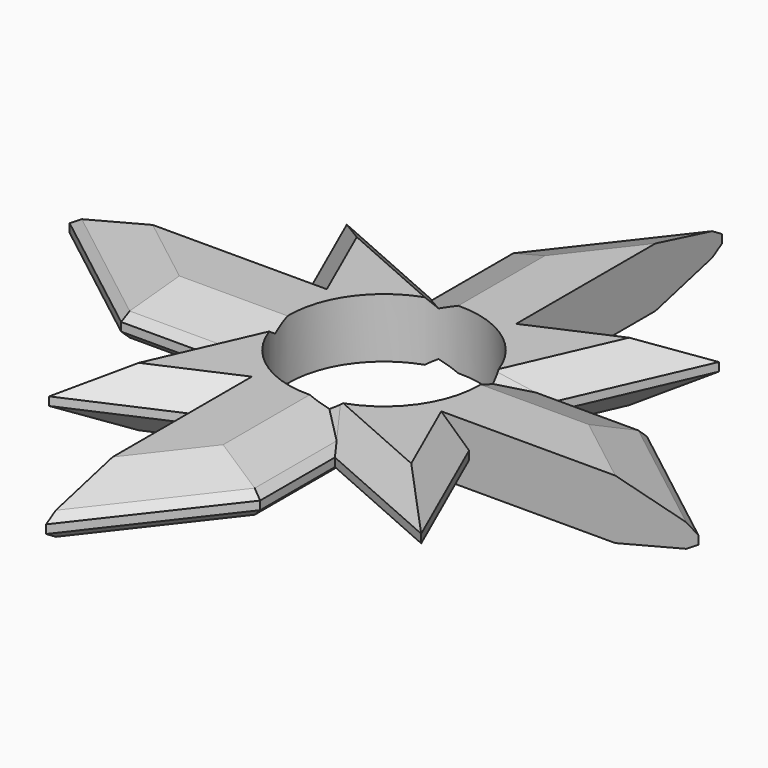
from build123d import *

# Parameters (mm, degrees)
F1_DEPTH      = 7
F2_T1_DEPTH   = 35.6796346597
F2_T3_DEPTH   = 35.6796346597
F2_T5_DEPTH   = 35.6796346597
F2_T7_DEPTH   = 35.6796346597
F2_T12_DEPTH  = 26.4420979278
F2_T17_DEPTH  = 26.4420979278
F2_T22_DEPTH  = 26.4420979278
F2_T27_DEPTH  = 26.4420979278
F2_T32_DEPTH  = 32.5914188112
F2_T37_DEPTH  = 32.5914188112
F2_T42_DEPTH  = 32.5914188112
F2_T47_DEPTH  = 32.5914188112
F2_T52_DEPTH  = 32.5914188112
F2_T57_DEPTH  = 32.5914188112
F2_T62_DEPTH  = 32.5914188112
F2_T67_DEPTH  = 32.5914188112
F2_T72_DEPTH  = 26.4420979278
F2_T77_DEPTH  = 32.5914188112
F2_T82_DEPTH  = 32.5914188112
F2_T87_DEPTH  = 26.4420979278
F2_T92_DEPTH  = 32.5914188112
F2_T97_DEPTH  = 32.5914188112
F2_T102_DEPTH = 26.4420979278
F2_T107_DEPTH = 32.5914188112
F2_T112_DEPTH = 32.5914188112
F2_T117_DEPTH = 26.4420979278
F2_T122_DEPTH = 32.5914188112
F2_T127_DEPTH = 32.5914188112
F2_T133_DEPTH = 26.4420979278
F2_T137_DEPTH = 32.5914188112
F2_T144_DEPTH = 26.4420979278
F2_T148_DEPTH = 32.5914188112
F2_T155_DEPTH = 26.4420979278
F2_T159_DEPTH = 32.5914188112
F2_T166_DEPTH = 26.4420979278
F2_T170_DEPTH = 32.5914188112
F2_T177_DEPTH = 26.4420979278
F2_T181_DEPTH = 32.5914188112
F2_T188_DEPTH = 26.4420979278
F2_T192_DEPTH = 32.5914188112
F2_T199_DEPTH = 26.4420979278
F2_T203_DEPTH = 32.5914188112
F2_T210_DEPTH = 26.4420979278
F2_T214_DEPTH = 32.5914188112
F3_T1_DEPTH   = 30.9109915853
F3_T3_DEPTH   = 30.9109915853
F3_T5_DEPTH   = 30.9109915853
F3_T7_DEPTH   = 30.9109915853
F3_T12_DEPTH  = 29.7913643174
F3_T17_DEPTH  = 29.7913643174
F3_T22_DEPTH  = 29.7913643174
F3_T27_DEPTH  = 29.7913643174
F3_T32_DEPTH  = 29.7913643174
F3_T37_DEPTH  = 29.7913643174
F3_T42_DEPTH  = 29.7913643174
F3_T47_DEPTH  = 29.7913643174


# Not quite as in the source:
# - a fillet or chamfer that OpenCascade refuses, or shapes differently, is made with other operations: its cross-section is extruded or revolved along the edge and cut away or added


with BuildPart() as f1:
    # F0 (on Top) → F1 (new body)
    with BuildSketch(Plane.XY):
        Polygon((-6.2057178847, 25.9939282815), (6.2057178847, 25.9939282815), (6.2057178847, 41.9939282815), align=None)
        Polygon((-6.2057178847, 25.9939282815), (-6.2057178847, 14.9819282815), (6.2057178847, 25.9939282815), align=None)
        Polygon((6.2057178847, 25.9939282815), (-6.2057178847, 14.9819282815), (6.2057178847, 14.9819282815), align=None)
        Polygon((21.9075315821, 21.9075315821), (6.2057178847, 14.9819282815), (10.5938230831, 10.5938230831), align=None)
        Polygon((21.9075315821, 21.9075315821), (10.5938230831, 10.5938230831), (14.9819282815, 6.2057178847), align=None)
        Polygon((25.9939282815, 6.2057178847), (14.9819282815, 6.2057178847), (25.9939282815, -6.2057178847), align=None)
        Polygon((14.9819282815, 6.2057178847), (14.9819282815, -6.2057178847), (25.9939282815, -6.2057178847), align=None)
        Polygon((25.9939282815, 6.2057178847), (25.9939282815, -6.2057178847), (41.9939282815, -6.2057178847), align=None)
        Polygon((10.5938230831, -10.5938230831), (6.2057178847, -14.9819282815), (21.9075315821, -21.9075315821), align=None)
        Polygon((-14.9819282815, 6.2057178847), (-14.9819282815, 0), (-14.9819282815, -6.2057178847), (-10.5938230831, -10.5938230831), (-6.2057178847, -14.9819282815), (6.2057178847, -14.9819282815), (10.5938230831, -10.5938230831), (14.9819282815, -6.2057178847), (14.9819282815, 6.2057178847), (10.5938230831, 10.5938230831), (6.2057178847, 14.9819282815), (-6.2057178847, 14.9819282815), (-10.5938230831, 10.5938230831), align=None)
        with BuildLine():
            ThreePointArc((-11.2, 0), (0, 11.2), (11.2, 0))
            ThreePointArc((11.2, 0), (0, -11.2), (-11.2, 0))
        make_face(mode=Mode.SUBTRACT)
        Polygon((-25.9939282815, -6.2057178847), (-25.9939282815, 6.2057178847), (-41.9939282815, 6.2057178847), align=None)
        Polygon((-25.9939282815, -6.2057178847), (-14.9819282815, -6.2057178847), (-25.9939282815, 6.2057178847), align=None)
        Polygon((-14.9819282815, -6.2057178847), (-14.9819282815, 0), (-14.9819282815, 6.2057178847), (-25.9939282815, 6.2057178847), align=None)
        Polygon((-21.9075315821, 21.9075315821), (-14.9819282815, 6.2057178847), (-10.5938230831, 10.5938230831), align=None)
        Polygon((-21.9075315821, 21.9075315821), (-10.5938230831, 10.5938230831), (-6.2057178847, 14.9819282815), align=None)
        Polygon((6.2057178847, -25.9939282815), (6.2057178847, -14.9819282815), (-6.2057178847, -25.9939282815), align=None)
        Polygon((6.2057178847, -25.9939282815), (-6.2057178847, -25.9939282815), (-6.2057178847, -41.9939282815), align=None)
        Polygon((6.2057178847, -14.9819282815), (-6.2057178847, -14.9819282815), (-6.2057178847, -25.9939282815), align=None)
        Polygon((-6.2057178847, -14.9819282815), (-10.5938230831, -10.5938230831), (-21.9075315821, -21.9075315821), align=None)
        Polygon((-10.5938230831, -10.5938230831), (-14.9819282815, -6.2057178847), (-21.9075315821, -21.9075315821), align=None)
        Polygon((14.9819282815, -6.2057178847), (10.5938230831, -10.5938230831), (21.9075315821, -21.9075315821), align=None)
    extrude(amount=F1_DEPTH)

    # F2: chamfer of 3 on 32 edges, made by hand

    # F2_s2 → F2_t1 (cut)
    with BuildSketch(Plane(origin=(27.3976190365, 35.3191937444, 0), x_dir=(0, 0, 1), z_dir=(-0.6129244305, -0.7901415332, 0))):
        Polygon((4, 20.8357091325), (7, 17.8357091325), (7, 20.8357091325), align=None)
        Polygon((3, 20.8357091325), (0, 17.8357091325), (0, 20.8357091325), align=None)
    extrude(amount=F2_T1_DEPTH, mode=Mode.SUBTRACT)

    # F2_s4 → F2_t3 (cut)
    with BuildSketch(Plane(origin=(-35.3191937444, 27.3976190365, 0), x_dir=(0, 0, 1), z_dir=(0.7901415332, -0.6129244305, 0))):
        Polygon((4, 20.8357091325), (7, 17.8357091325), (7, 20.8357091325), align=None)
        Polygon((3, 20.8357091325), (0, 17.8357091325), (0, 20.8357091325), align=None)
    extrude(amount=F2_T3_DEPTH, mode=Mode.SUBTRACT)

    # F2_s6 → F2_t5 (cut)
    with BuildSketch(Plane(origin=(-27.3976190365, -35.3191937444, 0), x_dir=(0, 0, 1), z_dir=(0.6129244305, 0.7901415332, 0))):
        Polygon((4, 20.8357091325), (7, 17.8357091325), (7, 20.8357091325), align=None)
        Polygon((3, 20.8357091325), (0, 17.8357091325), (0, 20.8357091325), align=None)
    extrude(amount=F2_T5_DEPTH, mode=Mode.SUBTRACT)

    # F2_s8 → F2_t7 (cut)
    with BuildSketch(Plane(origin=(35.3191937444, -27.3976190365, 0), x_dir=(0, 0, 1), z_dir=(-0.7901415332, 0.6129244305, 0))):
        Polygon((4, 20.8357091325), (7, 17.8357091325), (7, 20.8357091325), align=None)
        Polygon((3, 20.8357091325), (0, 17.8357091325), (0, 20.8357091325), align=None)
    extrude(amount=F2_T7_DEPTH, mode=Mode.SUBTRACT)


with BuildPart() as f2_tool10:
    # F2_s11 → F2_t12 (new body)
    with BuildSketch(Plane.YZ.offset(33.7089772454)):
        Polygon((6.2057178847, 4), (3.2057178847, 7), (6.2057178847, 7), align=None)
    extrude(amount=-F2_T12_DEPTH)

    split(bisect_by=Plane(origin=(10.2505901429, -4.5212306231, 0), x_dir=(0, 0, 1), z_dir=(0.9149536801, -0.4035588722, 0)), keep=Keep.TOP)


with BuildPart() as f1_1:
    add(f1.part)

    # F2_t9: cut F2_tool10
    add(f2_tool10.part, mode=Mode.SUBTRACT)


with BuildPart() as f2_tool15:
    # F2_s16 → F2_t17 (new body)
    with BuildSketch(Plane.XZ.offset(33.7089772454)):
        Polygon((6.2057178847, 4), (3.2057178847, 7), (6.2057178847, 7), align=None)
    extrude(amount=-F2_T17_DEPTH)

    split(bisect_by=Plane(origin=(-4.5212306231, -10.2505901429, 0), x_dir=(0, 0, 1), z_dir=(-0.4035588722, -0.9149536801, 0)), keep=Keep.TOP)


with BuildPart() as f1_2:
    add(f1_1.part)

    # F2_t14: cut F2_tool15
    add(f2_tool15.part, mode=Mode.SUBTRACT)


with BuildPart() as f2_tool20:
    # F2_s21 → F2_t22 (new body)
    with BuildSketch(Plane.YZ.offset(-33.7089772454)):
        Polygon((-6.2057178847, 4), (-3.2057178847, 7), (-6.2057178847, 7), align=None)
    extrude(amount=F2_T22_DEPTH)

    split(bisect_by=Plane(origin=(-10.2505901429, 4.5212306231, 0), x_dir=(0, 0, 1), z_dir=(-0.9149536801, 0.4035588722, 0)), keep=Keep.TOP)


with BuildPart() as f1_3:
    add(f1_2.part)

    # F2_t19: cut F2_tool20
    add(f2_tool20.part, mode=Mode.SUBTRACT)


with BuildPart() as f2_tool25:
    # F2_s26 → F2_t27 (new body)
    with BuildSketch(Plane.XZ.offset(-33.7089772454)):
        Polygon((-6.2057178847, 4), (-3.2057178847, 7), (-6.2057178847, 7), align=None)
    extrude(amount=F2_T27_DEPTH)

    split(bisect_by=Plane(origin=(4.5212306231, 10.2505901429, 0), x_dir=(0, 0, 1), z_dir=(0.4035588722, 0.9149536801, 0)), keep=Keep.TOP)


with BuildPart() as f1_4:
    add(f1_3.part)

    # F2_t24: cut F2_tool25
    add(f2_tool25.part, mode=Mode.SUBTRACT)


with BuildPart() as f2_tool30:
    # F2_s31 → F2_t32 (new body)
    with BuildSketch(Plane(origin=(-3.6680360663, 1.61786168, 0), x_dir=(0, 0, 1), z_dir=(-0.9149536801, 0.4035588722, 0))):
        Polygon((4, 11.2033979054), (7, 8.2033979054), (7, 11.2033979054), align=None)
    extrude(amount=F2_T32_DEPTH)

    split(bisect_by=Plane.YZ.offset(-6.2057178847), keep=Keep.BOTTOM)


with BuildPart() as f1_5:
    add(f1_4.part)

    # F2_t29: cut F2_tool30
    add(f2_tool30.part, mode=Mode.SUBTRACT)


with BuildPart() as f2_tool35:
    # F2_s36 → F2_t37 (new body)
    with BuildSketch(Plane(origin=(-14.7704178977, 33.4876746467, 0), x_dir=(0, 0, 1), z_dir=(0.4035588722, -0.9149536801, 0))):
        Polygon((4, 11.2033979054), (7, 8.2033979054), (7, 11.2033979054), align=None)
    extrude(amount=F2_T37_DEPTH)

    split(bisect_by=Plane.XZ.offset(-6.2057178847), keep=Keep.BOTTOM)


with BuildPart() as f1_6:
    add(f1_5.part)

    # F2_t34: cut F2_tool35
    add(f2_tool35.part, mode=Mode.SUBTRACT)


with BuildPart() as f2_tool40:
    # F2_s41 → F2_t42 (new body)
    with BuildSketch(Plane(origin=(33.4876746467, 14.7704178977, 0), x_dir=(0, 0, 1), z_dir=(-0.9149536801, -0.4035588722, 0))):
        Polygon((4, 11.2033979054), (7, 8.2033979054), (7, 11.2033979054), align=None)
    extrude(amount=F2_T42_DEPTH)

    split(bisect_by=Plane.YZ.offset(6.2057178847), keep=Keep.TOP)


with BuildPart() as f1_7:
    add(f1_6.part)

    # F2_t39: cut F2_tool40
    add(f2_tool40.part, mode=Mode.SUBTRACT)


with BuildPart() as f2_tool45:
    # F2_s46 → F2_t47 (new body)
    with BuildSketch(Plane(origin=(1.61786168, 3.6680360663, 0), x_dir=(0, 0, 1), z_dir=(0.4035588722, 0.9149536801, 0))):
        Polygon((4, 11.2033979054), (7, 8.2033979054), (7, 11.2033979054), align=None)
    extrude(amount=F2_T47_DEPTH)

    split(bisect_by=Plane.XZ.offset(-6.2057178847), keep=Keep.BOTTOM)


with BuildPart() as f1_8:
    add(f1_7.part)

    # F2_t44: cut F2_tool45
    add(f2_tool45.part, mode=Mode.SUBTRACT)


with BuildPart() as f2_tool50:
    # F2_s51 → F2_t52 (new body)
    with BuildSketch(Plane(origin=(-1.61786168, -3.6680360663, 0), x_dir=(0, 0, 1), z_dir=(-0.4035588722, -0.9149536801, 0))):
        Polygon((4, 11.2033979054), (7, 8.2033979054), (7, 11.2033979054), align=None)
    extrude(amount=F2_T52_DEPTH)

    split(bisect_by=Plane.XZ.offset(6.2057178847), keep=Keep.TOP)


with BuildPart() as f1_9:
    add(f1_8.part)

    # F2_t49: cut F2_tool50
    add(f2_tool50.part, mode=Mode.SUBTRACT)


with BuildPart() as f2_tool55:
    # F2_s56 → F2_t57 (new body)
    with BuildSketch(Plane(origin=(-33.4876746467, -14.7704178977, 0), x_dir=(0, 0, 1), z_dir=(0.9149536801, 0.4035588722, 0))):
        Polygon((4, 11.2033979054), (7, 8.2033979054), (7, 11.2033979054), align=None)
    extrude(amount=F2_T57_DEPTH)

    split(bisect_by=Plane.YZ.offset(-6.2057178847), keep=Keep.BOTTOM)


with BuildPart() as f1_10:
    add(f1_9.part)

    # F2_t54: cut F2_tool55
    add(f2_tool55.part, mode=Mode.SUBTRACT)


with BuildPart() as f2_tool60:
    # F2_s61 → F2_t62 (new body)
    with BuildSketch(Plane(origin=(3.6680360663, -1.61786168, 0), x_dir=(0, 0, 1), z_dir=(0.9149536801, -0.4035588722, 0))):
        Polygon((4, 11.2033979054), (7, 8.2033979054), (7, 11.2033979054), align=None)
    extrude(amount=F2_T62_DEPTH)

    split(bisect_by=Plane.YZ.offset(6.2057178847), keep=Keep.TOP)


with BuildPart() as f1_11:
    add(f1_10.part)

    # F2_t59: cut F2_tool60
    add(f2_tool60.part, mode=Mode.SUBTRACT)


with BuildPart() as f2_tool65:
    # F2_s66 → F2_t67 (new body)
    with BuildSketch(Plane(origin=(14.7704178977, -33.4876746467, 0), x_dir=(0, 0, 1), z_dir=(-0.4035588722, 0.9149536801, 0))):
        Polygon((4, 11.2033979054), (7, 8.2033979054), (7, 11.2033979054), align=None)
    extrude(amount=F2_T67_DEPTH)

    split(bisect_by=Plane.XZ.offset(6.2057178847), keep=Keep.TOP)


with BuildPart() as f1_12:
    add(f1_11.part)

    # F2_t64: cut F2_tool65
    add(f2_tool65.part, mode=Mode.SUBTRACT)


with BuildPart() as f2_tool70:
    # F2_s71 → F2_t72 (new body)
    with BuildSketch(Plane.YZ.offset(33.7089772454)):
        Polygon((6.2057178847, 3), (3.2057178847, 0), (6.2057178847, 0), align=None)
    extrude(amount=-F2_T72_DEPTH)

    split(bisect_by=Plane(origin=(10.2505901429, -4.5212306231, 0), x_dir=(0, 0, 1), z_dir=(0.9149536801, -0.4035588722, 0)), keep=Keep.TOP)


with BuildPart() as f1_13:
    add(f1_12.part)

    # F2_t69: cut F2_tool70
    add(f2_tool70.part, mode=Mode.SUBTRACT)


with BuildPart() as f2_tool75:
    # F2_s76 → F2_t77 (new body)
    with BuildSketch(Plane(origin=(1.61786168, 3.6680360663, 0), x_dir=(0, 0, 1), z_dir=(0.4035588722, 0.9149536801, 0))):
        Polygon((3, 11.2033979054), (0, 8.2033979054), (0, 11.2033979054), align=None)
    extrude(amount=F2_T77_DEPTH)

    split(bisect_by=Plane.XZ.offset(-6.2057178847), keep=Keep.BOTTOM)


with BuildPart() as f1_14:
    add(f1_13.part)

    # F2_t74: cut F2_tool75
    add(f2_tool75.part, mode=Mode.SUBTRACT)


with BuildPart() as f2_tool80:
    # F2_s81 → F2_t82 (new body)
    with BuildSketch(Plane(origin=(33.4876746467, 14.7704178977, 0), x_dir=(0, 0, 1), z_dir=(-0.9149536801, -0.4035588722, 0))):
        Polygon((3, 11.2033979054), (0, 8.2033979054), (0, 11.2033979054), align=None)
    extrude(amount=F2_T82_DEPTH)

    split(bisect_by=Plane.YZ.offset(6.2057178847), keep=Keep.TOP)


with BuildPart() as f1_15:
    add(f1_14.part)

    # F2_t79: cut F2_tool80
    add(f2_tool80.part, mode=Mode.SUBTRACT)


with BuildPart() as f2_tool85:
    # F2_s86 → F2_t87 (new body)
    with BuildSketch(Plane.XZ.offset(-33.7089772454)):
        Polygon((-6.2057178847, 3), (-3.2057178847, 0), (-6.2057178847, 0), align=None)
    extrude(amount=F2_T87_DEPTH)

    split(bisect_by=Plane(origin=(4.5212306231, 10.2505901429, 0), x_dir=(0, 0, 1), z_dir=(0.4035588722, 0.9149536801, 0)), keep=Keep.TOP)


with BuildPart() as f1_16:
    add(f1_15.part)

    # F2_t84: cut F2_tool85
    add(f2_tool85.part, mode=Mode.SUBTRACT)


with BuildPart() as f2_tool90:
    # F2_s91 → F2_t92 (new body)
    with BuildSketch(Plane(origin=(-3.6680360663, 1.61786168, 0), x_dir=(0, 0, 1), z_dir=(-0.9149536801, 0.4035588722, 0))):
        Polygon((3, 11.2033979054), (0, 8.2033979054), (0, 11.2033979054), align=None)
    extrude(amount=F2_T92_DEPTH)

    split(bisect_by=Plane.YZ.offset(-6.2057178847), keep=Keep.BOTTOM)


with BuildPart() as f1_17:
    add(f1_16.part)

    # F2_t89: cut F2_tool90
    add(f2_tool90.part, mode=Mode.SUBTRACT)


with BuildPart() as f2_tool95:
    # F2_s96 → F2_t97 (new body)
    with BuildSketch(Plane(origin=(-14.7704178977, 33.4876746467, 0), x_dir=(0, 0, 1), z_dir=(0.4035588722, -0.9149536801, 0))):
        Polygon((3, 11.2033979054), (0, 8.2033979054), (0, 11.2033979054), align=None)
    extrude(amount=F2_T97_DEPTH)

    split(bisect_by=Plane.XZ.offset(-6.2057178847), keep=Keep.BOTTOM)


with BuildPart() as f1_18:
    add(f1_17.part)

    # F2_t94: cut F2_tool95
    add(f2_tool95.part, mode=Mode.SUBTRACT)


with BuildPart() as f2_tool100:
    # F2_s101 → F2_t102 (new body)
    with BuildSketch(Plane.YZ.offset(-33.7089772454)):
        Polygon((-6.2057178847, 3), (-3.2057178847, 0), (-6.2057178847, 0), align=None)
    extrude(amount=F2_T102_DEPTH)

    split(bisect_by=Plane(origin=(-10.2505901429, 4.5212306231, 0), x_dir=(0, 0, 1), z_dir=(-0.9149536801, 0.4035588722, 0)), keep=Keep.TOP)


with BuildPart() as f1_19:
    add(f1_18.part)

    # F2_t99: cut F2_tool100
    add(f2_tool100.part, mode=Mode.SUBTRACT)


with BuildPart() as f2_tool105:
    # F2_s106 → F2_t107 (new body)
    with BuildSketch(Plane(origin=(-1.61786168, -3.6680360663, 0), x_dir=(0, 0, 1), z_dir=(-0.4035588722, -0.9149536801, 0))):
        Polygon((3, 11.2033979054), (0, 8.2033979054), (0, 11.2033979054), align=None)
    extrude(amount=F2_T107_DEPTH)

    split(bisect_by=Plane.XZ.offset(6.2057178847), keep=Keep.TOP)


with BuildPart() as f1_20:
    add(f1_19.part)

    # F2_t104: cut F2_tool105
    add(f2_tool105.part, mode=Mode.SUBTRACT)


with BuildPart() as f2_tool110:
    # F2_s111 → F2_t112 (new body)
    with BuildSketch(Plane(origin=(-33.4876746467, -14.7704178977, 0), x_dir=(0, 0, 1), z_dir=(0.9149536801, 0.4035588722, 0))):
        Polygon((3, 11.2033979054), (0, 8.2033979054), (0, 11.2033979054), align=None)
    extrude(amount=F2_T112_DEPTH)

    split(bisect_by=Plane.YZ.offset(-6.2057178847), keep=Keep.BOTTOM)


with BuildPart() as f1_21:
    add(f1_20.part)

    # F2_t109: cut F2_tool110
    add(f2_tool110.part, mode=Mode.SUBTRACT)


with BuildPart() as f2_tool115:
    # F2_s116 → F2_t117 (new body)
    with BuildSketch(Plane.XZ.offset(33.7089772454)):
        Polygon((6.2057178847, 3), (3.2057178847, 0), (6.2057178847, 0), align=None)
    extrude(amount=-F2_T117_DEPTH)

    split(bisect_by=Plane(origin=(-4.5212306231, -10.2505901429, 0), x_dir=(0, 0, 1), z_dir=(-0.4035588722, -0.9149536801, 0)), keep=Keep.TOP)


with BuildPart() as f1_22:
    add(f1_21.part)

    # F2_t114: cut F2_tool115
    add(f2_tool115.part, mode=Mode.SUBTRACT)


with BuildPart() as f2_tool120:
    # F2_s121 → F2_t122 (new body)
    with BuildSketch(Plane(origin=(14.7704178977, -33.4876746467, 0), x_dir=(0, 0, 1), z_dir=(-0.4035588722, 0.9149536801, 0))):
        Polygon((3, 11.2033979054), (0, 8.2033979054), (0, 11.2033979054), align=None)
    extrude(amount=F2_T122_DEPTH)

    split(bisect_by=Plane.XZ.offset(6.2057178847), keep=Keep.TOP)


with BuildPart() as f1_23:
    add(f1_22.part)

    # F2_t119: cut F2_tool120
    add(f2_tool120.part, mode=Mode.SUBTRACT)


with BuildPart() as f2_tool125:
    # F2_s126 → F2_t127 (new body)
    with BuildSketch(Plane(origin=(3.6680360663, -1.61786168, 0), x_dir=(0, 0, 1), z_dir=(0.9149536801, -0.4035588722, 0))):
        Polygon((3, 11.2033979054), (0, 8.2033979054), (0, 11.2033979054), align=None)
    extrude(amount=F2_T127_DEPTH)

    split(bisect_by=Plane.YZ.offset(6.2057178847), keep=Keep.TOP)


with BuildPart() as f1_24:
    add(f1_23.part)

    # F2_t124: cut F2_tool125
    add(f2_tool125.part, mode=Mode.SUBTRACT)


with BuildPart() as f2_tool131:
    # F2_s132 → F2_t133 (new body)
    with BuildSketch(Plane.YZ.offset(33.7089772454)):
        Polygon((6.2057178847, 4), (3.2057178847, 7), (6.2057178847, 7), align=None)
    extrude(amount=-F2_T133_DEPTH)

    split(bisect_by=Plane(origin=(10.2505901429, -4.5212306231, 0), x_dir=(0, 0, 1), z_dir=(-0.9149536801, 0.4035588722, 0)), keep=Keep.TOP)


with BuildPart() as f2_tool135:
    # F2_s136 → F2_t137 (new body)
    with BuildSketch(Plane(origin=(1.61786168, 3.6680360663, 0), x_dir=(0, 0, 1), z_dir=(0.4035588722, 0.9149536801, 0))):
        Polygon((4, 11.2033979054), (7, 8.2033979054), (7, 11.2033979054), align=None)
    extrude(amount=F2_T137_DEPTH)

    split(bisect_by=Plane.XZ.offset(-6.2057178847), keep=Keep.TOP)


with BuildPart() as f2_tool131_1:
    add(f2_tool131.part)

    # F2_t139: intersect F2_tool135
    add(f2_tool135.part, mode=Mode.INTERSECT)


with BuildPart() as f1_25:
    add(f1_24.part)

    # F2_t129: cut F2_tool131
    add(f2_tool131_1.part, mode=Mode.SUBTRACT)


with BuildPart() as f2_tool142:
    # F2_s143 → F2_t144 (new body)
    with BuildSketch(Plane.XZ.offset(33.7089772454)):
        Polygon((6.2057178847, 4), (3.2057178847, 7), (6.2057178847, 7), align=None)
    extrude(amount=-F2_T144_DEPTH)

    split(bisect_by=Plane(origin=(-4.5212306231, -10.2505901429, 0), x_dir=(0, 0, 1), z_dir=(0.4035588722, 0.9149536801, 0)), keep=Keep.TOP)


with BuildPart() as f2_tool146:
    # F2_s147 → F2_t148 (new body)
    with BuildSketch(Plane(origin=(3.6680360663, -1.61786168, 0), x_dir=(0, 0, 1), z_dir=(0.9149536801, -0.4035588722, 0))):
        Polygon((4, 11.2033979054), (7, 8.2033979054), (7, 11.2033979054), align=None)
    extrude(amount=F2_T148_DEPTH)

    split(bisect_by=Plane.YZ.offset(6.2057178847), keep=Keep.BOTTOM)


with BuildPart() as f2_tool142_1:
    add(f2_tool142.part)

    # F2_t150: intersect F2_tool146
    add(f2_tool146.part, mode=Mode.INTERSECT)


with BuildPart() as f1_26:
    add(f1_25.part)

    # F2_t140: cut F2_tool142
    add(f2_tool142_1.part, mode=Mode.SUBTRACT)


with BuildPart() as f2_tool153:
    # F2_s154 → F2_t155 (new body)
    with BuildSketch(Plane.YZ.offset(-33.7089772454)):
        Polygon((-6.2057178847, 4), (-3.2057178847, 7), (-6.2057178847, 7), align=None)
    extrude(amount=F2_T155_DEPTH)

    split(bisect_by=Plane(origin=(-10.2505901429, 4.5212306231, 0), x_dir=(0, 0, 1), z_dir=(0.9149536801, -0.4035588722, 0)), keep=Keep.TOP)


with BuildPart() as f2_tool157:
    # F2_s158 → F2_t159 (new body)
    with BuildSketch(Plane(origin=(-1.61786168, -3.6680360663, 0), x_dir=(0, 0, 1), z_dir=(-0.4035588722, -0.9149536801, 0))):
        Polygon((4, 11.2033979054), (7, 8.2033979054), (7, 11.2033979054), align=None)
    extrude(amount=F2_T159_DEPTH)

    split(bisect_by=Plane.XZ.offset(6.2057178847), keep=Keep.BOTTOM)


with BuildPart() as f2_tool153_1:
    add(f2_tool153.part)

    # F2_t161: intersect F2_tool157
    add(f2_tool157.part, mode=Mode.INTERSECT)


with BuildPart() as f1_27:
    add(f1_26.part)

    # F2_t151: cut F2_tool153
    add(f2_tool153_1.part, mode=Mode.SUBTRACT)


with BuildPart() as f2_tool164:
    # F2_s165 → F2_t166 (new body)
    with BuildSketch(Plane.XZ.offset(-33.7089772454)):
        Polygon((-6.2057178847, 4), (-3.2057178847, 7), (-6.2057178847, 7), align=None)
    extrude(amount=F2_T166_DEPTH)

    split(bisect_by=Plane(origin=(4.5212306231, 10.2505901429, 0), x_dir=(0, 0, 1), z_dir=(-0.4035588722, -0.9149536801, 0)), keep=Keep.TOP)


with BuildPart() as f2_tool168:
    # F2_s169 → F2_t170 (new body)
    with BuildSketch(Plane(origin=(-3.6680360663, 1.61786168, 0), x_dir=(0, 0, 1), z_dir=(-0.9149536801, 0.4035588722, 0))):
        Polygon((4, 11.2033979054), (7, 8.2033979054), (7, 11.2033979054), align=None)
    extrude(amount=F2_T170_DEPTH)

    split(bisect_by=Plane.YZ.offset(-6.2057178847), keep=Keep.TOP)


with BuildPart() as f2_tool164_1:
    add(f2_tool164.part)

    # F2_t172: intersect F2_tool168
    add(f2_tool168.part, mode=Mode.INTERSECT)


with BuildPart() as f1_28:
    add(f1_27.part)

    # F2_t162: cut F2_tool164
    add(f2_tool164_1.part, mode=Mode.SUBTRACT)


with BuildPart() as f2_tool175:
    # F2_s176 → F2_t177 (new body)
    with BuildSketch(Plane.YZ.offset(33.7089772454)):
        Polygon((6.2057178847, 3), (3.2057178847, 0), (6.2057178847, 0), align=None)
    extrude(amount=-F2_T177_DEPTH)

    split(bisect_by=Plane(origin=(10.2505901429, -4.5212306231, 0), x_dir=(0, 0, 1), z_dir=(-0.9149536801, 0.4035588722, 0)), keep=Keep.TOP)


with BuildPart() as f2_tool179:
    # F2_s180 → F2_t181 (new body)
    with BuildSketch(Plane(origin=(1.61786168, 3.6680360663, 0), x_dir=(0, 0, 1), z_dir=(0.4035588722, 0.9149536801, 0))):
        Polygon((3, 11.2033979054), (0, 8.2033979054), (0, 11.2033979054), align=None)
    extrude(amount=F2_T181_DEPTH)

    split(bisect_by=Plane.XZ.offset(-6.2057178847), keep=Keep.TOP)


with BuildPart() as f2_tool175_1:
    add(f2_tool175.part)

    # F2_t183: intersect F2_tool179
    add(f2_tool179.part, mode=Mode.INTERSECT)


with BuildPart() as f1_29:
    add(f1_28.part)

    # F2_t173: cut F2_tool175
    add(f2_tool175_1.part, mode=Mode.SUBTRACT)


with BuildPart() as f2_tool186:
    # F2_s187 → F2_t188 (new body)
    with BuildSketch(Plane.XZ.offset(-33.7089772454)):
        Polygon((-6.2057178847, 3), (-3.2057178847, 0), (-6.2057178847, 0), align=None)
    extrude(amount=F2_T188_DEPTH)

    split(bisect_by=Plane(origin=(4.5212306231, 10.2505901429, 0), x_dir=(0, 0, 1), z_dir=(-0.4035588722, -0.9149536801, 0)), keep=Keep.TOP)


with BuildPart() as f2_tool190:
    # F2_s191 → F2_t192 (new body)
    with BuildSketch(Plane(origin=(-3.6680360663, 1.61786168, 0), x_dir=(0, 0, 1), z_dir=(-0.9149536801, 0.4035588722, 0))):
        Polygon((3, 11.2033979054), (0, 8.2033979054), (0, 11.2033979054), align=None)
    extrude(amount=F2_T192_DEPTH)

    split(bisect_by=Plane.YZ.offset(-6.2057178847), keep=Keep.TOP)


with BuildPart() as f2_tool186_1:
    add(f2_tool186.part)

    # F2_t194: intersect F2_tool190
    add(f2_tool190.part, mode=Mode.INTERSECT)


with BuildPart() as f1_30:
    add(f1_29.part)

    # F2_t184: cut F2_tool186
    add(f2_tool186_1.part, mode=Mode.SUBTRACT)


with BuildPart() as f2_tool197:
    # F2_s198 → F2_t199 (new body)
    with BuildSketch(Plane.YZ.offset(-33.7089772454)):
        Polygon((-6.2057178847, 3), (-3.2057178847, 0), (-6.2057178847, 0), align=None)
    extrude(amount=F2_T199_DEPTH)

    split(bisect_by=Plane(origin=(-10.2505901429, 4.5212306231, 0), x_dir=(0, 0, 1), z_dir=(0.9149536801, -0.4035588722, 0)), keep=Keep.TOP)


with BuildPart() as f2_tool201:
    # F2_s202 → F2_t203 (new body)
    with BuildSketch(Plane(origin=(-1.61786168, -3.6680360663, 0), x_dir=(0, 0, 1), z_dir=(-0.4035588722, -0.9149536801, 0))):
        Polygon((3, 11.2033979054), (0, 8.2033979054), (0, 11.2033979054), align=None)
    extrude(amount=F2_T203_DEPTH)

    split(bisect_by=Plane.XZ.offset(6.2057178847), keep=Keep.BOTTOM)


with BuildPart() as f2_tool197_1:
    add(f2_tool197.part)

    # F2_t205: intersect F2_tool201
    add(f2_tool201.part, mode=Mode.INTERSECT)


with BuildPart() as f1_31:
    add(f1_30.part)

    # F2_t195: cut F2_tool197
    add(f2_tool197_1.part, mode=Mode.SUBTRACT)


with BuildPart() as f2_tool208:
    # F2_s209 → F2_t210 (new body)
    with BuildSketch(Plane.XZ.offset(33.7089772454)):
        Polygon((6.2057178847, 3), (3.2057178847, 0), (6.2057178847, 0), align=None)
    extrude(amount=-F2_T210_DEPTH)

    split(bisect_by=Plane(origin=(-4.5212306231, -10.2505901429, 0), x_dir=(0, 0, 1), z_dir=(0.4035588722, 0.9149536801, 0)), keep=Keep.TOP)


with BuildPart() as f2_tool212:
    # F2_s213 → F2_t214 (new body)
    with BuildSketch(Plane(origin=(3.6680360663, -1.61786168, 0), x_dir=(0, 0, 1), z_dir=(0.9149536801, -0.4035588722, 0))):
        Polygon((3, 11.2033979054), (0, 8.2033979054), (0, 11.2033979054), align=None)
    extrude(amount=F2_T214_DEPTH)

    split(bisect_by=Plane.YZ.offset(6.2057178847), keep=Keep.BOTTOM)


with BuildPart() as f2_tool208_1:
    add(f2_tool208.part)

    # F2_t216: intersect F2_tool212
    add(f2_tool212.part, mode=Mode.INTERSECT)


with BuildPart() as f1_32:
    add(f1_31.part)

    # F2_t206: cut F2_tool208
    add(f2_tool208_1.part, mode=Mode.SUBTRACT)

    # F3: chamfer of 3 on 16 edges, made by hand

    # F3_s2 → F3_t1 (cut)
    with BuildSketch(Plane(origin=(-25.0657855166, -32.3131485927, 0), x_dir=(0, 0, 1), z_dir=(0.6129244305, 0.7901415332, 0))):
        Polygon((2.1213203436, 19.9570294761), (0, 14.8357091325), (0, 17.8357091325), align=None)
        Polygon((4.8786796564, 19.9570294761), (7, 14.8357091325), (7, 17.8357091325), align=None)
    extrude(amount=F3_T1_DEPTH, mode=Mode.SUBTRACT)

    # F3_s4 → F3_t3 (cut)
    with BuildSketch(Plane(origin=(-32.3131485927, 25.0657855166, 0), x_dir=(0, 0, 1), z_dir=(0.7901415332, -0.6129244305, 0))):
        Polygon((2.1213203436, 19.9570294761), (0, 14.8357091325), (0, 17.8357091325), align=None)
        Polygon((4.8786796564, 19.9570294761), (7, 14.8357091325), (7, 17.8357091325), align=None)
    extrude(amount=F3_T3_DEPTH, mode=Mode.SUBTRACT)

    # F3_s6 → F3_t5 (cut)
    with BuildSketch(Plane(origin=(25.0657855166, 32.3131485927, 0), x_dir=(0, 0, 1), z_dir=(-0.6129244305, -0.7901415332, 0))):
        Polygon((0, 14.8357091325), (2.1213203436, 19.9570294761), (0, 17.8357091325), align=None)
        Polygon((7, 14.8357091325), (4.8786796564, 19.9570294761), (7, 17.8357091325), align=None)
    extrude(amount=F3_T5_DEPTH, mode=Mode.SUBTRACT)

    # F3_s8 → F3_t7 (cut)
    with BuildSketch(Plane(origin=(32.3131485927, -25.0657855166, 0), x_dir=(0, 0, 1), z_dir=(-0.7901415332, 0.6129244305, 0))):
        Polygon((2.1213203436, 19.9570294761), (0, 14.8357091325), (0, 17.8357091325), align=None)
        Polygon((4.8786796564, 19.9570294761), (7, 14.8357091325), (7, 17.8357091325), align=None)
    extrude(amount=F3_T7_DEPTH, mode=Mode.SUBTRACT)


with BuildPart() as f3_tool10:
    # F3_s11 → F3_t12 (new body)
    with BuildSketch(Plane.XZ.offset(32.7447730281)):
        Polygon((5.3270382283, 2.1213203436), (0.2057178847, 0), (3.2057178847, 0), align=None)
    extrude(amount=-F3_T12_DEPTH)

    split(bisect_by=Plane(origin=(-1.6552770033, -3.7528645514, -4.1016989527), x_dir=(0.9149536801, -0.4035588722, 0), z_dir=(-0.2853592151, -0.6469699517, -0.7071067812)), keep=Keep.TOP)


with BuildPart() as f1_33:
    add(f1_32.part)

    # F3_t9: cut F3_tool10
    add(f3_tool10.part, mode=Mode.SUBTRACT)


with BuildPart() as f3_tool15:
    # F3_s16 → F3_t17 (new body)
    with BuildSketch(Plane.YZ.offset(-32.7447730281)):
        Polygon((-5.3270382283, 2.1213203436), (-0.2057178847, 0), (-3.2057178847, 0), align=None)
    extrude(amount=F3_T17_DEPTH)

    split(bisect_by=Plane(origin=(-3.7528645514, 1.6552770033, -4.1016989527), x_dir=(-0.4035588722, -0.9149536801, 0), z_dir=(-0.6469699517, 0.2853592151, -0.7071067812)), keep=Keep.TOP)


with BuildPart() as f1_34:
    add(f1_33.part)

    # F3_t14: cut F3_tool15
    add(f3_tool15.part, mode=Mode.SUBTRACT)


with BuildPart() as f3_tool20:
    # F3_s21 → F3_t22 (new body)
    with BuildSketch(Plane.XZ.offset(-2.9534087107)):
        Polygon((-5.3270382283, 2.1213203436), (-0.2057178847, 0), (-3.2057178847, 0), align=None)
    extrude(amount=-F3_T22_DEPTH)

    split(bisect_by=Plane(origin=(1.6552770033, 3.7528645514, -4.1016989527), x_dir=(-0.9149536801, 0.4035588722, 0), z_dir=(0.2853592151, 0.6469699517, -0.7071067812)), keep=Keep.TOP)


with BuildPart() as f1_35:
    add(f1_34.part)

    # F3_t19: cut F3_tool20
    add(f3_tool20.part, mode=Mode.SUBTRACT)


with BuildPart() as f3_tool25:
    # F3_s26 → F3_t27 (new body)
    with BuildSketch(Plane.YZ.offset(2.9534087107)):
        Polygon((5.3270382283, 2.1213203436), (0.2057178847, 0), (3.2057178847, 0), align=None)
    extrude(amount=F3_T27_DEPTH)

    split(bisect_by=Plane(origin=(3.7528645514, -1.6552770033, -4.1016989527), x_dir=(0.4035588722, 0.9149536801, 0), z_dir=(0.6469699517, -0.2853592151, -0.7071067812)), keep=Keep.TOP)


with BuildPart() as f1_36:
    add(f1_35.part)

    # F3_t24: cut F3_tool25
    add(f3_tool25.part, mode=Mode.SUBTRACT)


with BuildPart() as f3_tool30:
    # F3_s31 → F3_t32 (new body)
    with BuildSketch(Plane.XZ.offset(-2.9534087107)):
        Polygon((-0.2057178847, 7), (-5.3270382283, 4.8786796564), (-3.2057178847, 7), align=None)
    extrude(amount=-F3_T32_DEPTH)

    split(bisect_by=Plane(origin=(3.0677330559, 6.9552024317, 7.6016989527), x_dir=(-0.9149536801, 0.4035588722, 0), z_dir=(0.2853592151, 0.6469699517, 0.7071067812)), keep=Keep.TOP)


with BuildPart() as f1_37:
    add(f1_36.part)

    # F3_t29: cut F3_tool30
    add(f3_tool30.part, mode=Mode.SUBTRACT)


with BuildPart() as f3_tool35:
    # F3_s36 → F3_t37 (new body)
    with BuildSketch(Plane.YZ.offset(-32.7447730281)):
        Polygon((-0.2057178847, 7), (-5.3270382283, 4.8786796564), (-3.2057178847, 7), align=None)
    extrude(amount=F3_T37_DEPTH)

    split(bisect_by=Plane(origin=(-6.9552024317, 3.0677330559, 7.6016989527), x_dir=(-0.4035588722, -0.9149536801, 0), z_dir=(-0.6469699517, 0.2853592151, 0.7071067812)), keep=Keep.TOP)


with BuildPart() as f1_38:
    add(f1_37.part)

    # F3_t34: cut F3_tool35
    add(f3_tool35.part, mode=Mode.SUBTRACT)


with BuildPart() as f3_tool40:
    # F3_s41 → F3_t42 (new body)
    with BuildSketch(Plane.YZ.offset(32.7447730281)):
        Polygon((0.2057178847, 7), (5.3270382283, 4.8786796564), (3.2057178847, 7), align=None)
    extrude(amount=-F3_T42_DEPTH)

    split(bisect_by=Plane(origin=(6.9552024317, -3.0677330559, 7.6016989527), x_dir=(0.4035588722, 0.9149536801, 0), z_dir=(0.6469699517, -0.2853592151, 0.7071067812)), keep=Keep.TOP)


with BuildPart() as f1_39:
    add(f1_38.part)

    # F3_t39: cut F3_tool40
    add(f3_tool40.part, mode=Mode.SUBTRACT)


with BuildPart() as f3_tool45:
    # F3_s46 → F3_t47 (new body)
    with BuildSketch(Plane.XZ.offset(32.7447730281)):
        Polygon((0.2057178847, 7), (5.3270382283, 4.8786796564), (3.2057178847, 7), align=None)
    extrude(amount=-F3_T47_DEPTH)

    split(bisect_by=Plane(origin=(-3.0677330559, -6.9552024317, 7.6016989527), x_dir=(0.9149536801, -0.4035588722, 0), z_dir=(-0.2853592151, -0.6469699517, 0.7071067812)), keep=Keep.TOP)


with BuildPart() as f1_40:
    add(f1_39.part)

    # F3_t44: cut F3_tool45
    add(f3_tool45.part, mode=Mode.SUBTRACT)


solid = f1_40.part
